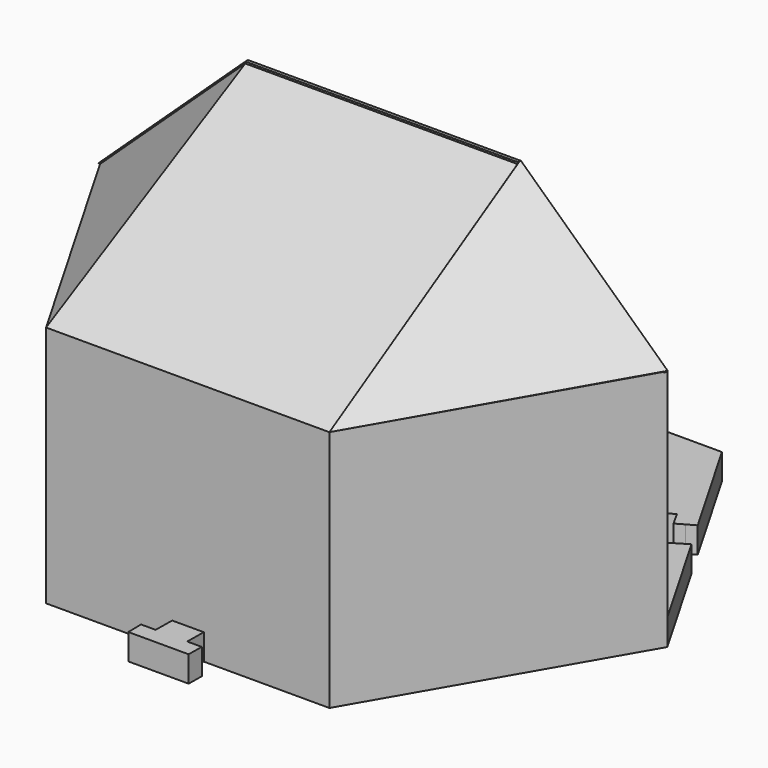
from build123d import *

# Parameters (mm, degrees)
F0_W      = 50
F0_H      = 12.5
F1_DEPTH  = 8
F2_DEPTH  = 75
F4_DEPTH  = 8
F7_DEPTH  = 3
F8_DEPTH  = 1
F11_DEPTH = 3
F14_DEPTH = 3
F15_DEPTH = 8
F16_DEPTH = 25
F17_DEPTH = 8
F18_DEPTH = 8
F19_DEPTH = 8


# Not quite as in the source:
# - a feature names something its author has since deleted; it is built from what else it names


with BuildPart() as f1:
    # F0 (on Top) → F1 (new body)
    with BuildSketch(Plane.XY):
        Polygon((-42.0179491924, 72.7772228311), (-60.5095952989, 40.7487522591), (-57.9695070384, 39.3207329262), (-55.5194165334, 43.6791064608), (-50.2642610162, 40.7248836223), (-52.7144317239, 36.366367418), (-57.615009792, 27.6494680496), (-60.0654171506, 23.2910848888), (-65.3204122546, 26.2455930623), (-62.870004896, 30.6039762231), (-65.5097997054, 32.0881441788), (-84.0358983849, 0), (-42.0179491924, -72.7772228311), (42.0179491924, -72.7772228311), (84.0358983849, 0), (65.5442522784, 32.028470572), (63.0375071287, 30.542699277), (65.5869240764, 26.2416718908), (60.4009142911, 23.1676851313), (60.2621924773, 23.4017175915), (60.0654171506, 23.2910848888), (57.615009792, 27.6494680496), (55.164720758, 32.0079177338), (52.8483970279, 36.1280767392), (52.7526466281, 36.0713280944), (50.2033797707, 40.372634697), (50.3975781651, 40.4877307774), (50.2642610162, 40.7248836223), (55.5194165334, 43.6791064608), (57.9695070384, 39.3207329262), (60.5095952989, 40.7487522591), (42.0179491924, 72.7772228311), align=None)
        with Locations((0, 54.5829171234)):
            Rectangle(F0_W, F0_H, mode=Mode.SUBTRACT)
    extrude(amount=F1_DEPTH)

    # F0 (on Top) → F2 (join)
    with BuildSketch(Plane.XY):
        Polygon((-84.0358983849, 0), (-87.5, 0), (-43.75, -75.7772228311), (-4.799692811, -75.7772228311), (4.9533583678, -75.7772228311), (43.75, -75.7772228311), (87.5, 0), (84.0358983849, 0), (42.0179491924, -72.7772228311), (-42.0179491924, -72.7772228311), align=None)
    extrude(amount=F2_DEPTH)

    # F0 (on Top) → F4 (join)
    with BuildSketch(Plane.XY):
        Polygon((43.75, 75.7772228311), (-43.75, 75.7772228311), (-63.1248363216, 42.2190219338), (-60.5095952989, 40.7487522591), (-42.0179491924, 72.7772228311), (42.0179491924, 72.7772228311), (60.5095952989, 40.7487522591), (63.1248363216, 42.2190219338), align=None)
    extrude(amount=F4_DEPTH)

    # F6 (on face) → F7 (join)
    with BuildSketch(Plane(origin=(0, -50.1312366318, 89.3836679776), x_dir=(1, 0, 0), z_dir=(0, 0.4891706574, -0.872188092))):
        Polygon((43.75, 29.4041920927), (0, 29.4041920927), (-43.75, 29.4041920927), (-42.01795, -57.4775522498), (42.01795, -57.4775522498), align=None)
    extrude(amount=F7_DEPTH)

    # F3 (on Front) → F8 (join)
    with BuildSketch(Plane.XZ):
        Polygon((-42.01795, 114.5), (0, 114.5), (42.01795, 114.5), (84.0359, 75), (87.5, 75), (42.01795, 117.5), (0, 117.5), (-42.01795, 117.5), (-87.5, 75), (-84.0359, 75), align=None)
    extrude(amount=F8_DEPTH)

    # F10 (on face) → F11 (join)
    with BuildSketch(Plane(origin=(-67.6846727043, -39.0777640058, 72.4338274863), x_dir=(0.7723629594, -0.3015876344, 0.5590173143), z_dir=(-0.6351814378, -0.3667221741, 0.6797495039))):
        Polygon((33.2314262259, 55.789645187), (-25.6554603702, 35.6104118215), (30.9888924807, -31.0804218073), align=None)
    extrude(amount=-F11_DEPTH)

    # F13 (on face) → F14 (join)
    with BuildSketch(Plane(origin=(67.6756688636, -39.5950852503, 72.4241918832), x_dir=(0.7733047167, 0.3041472681, -0.556322078), z_dir=(-0.6340345536, 0.3709553614, -0.6785221475))):
        Polygon((-30.939509805, 30.5117392321), (-32.8751652468, -56.3649154418), (25.9400068576, -35.9776056011), align=None)
    extrude(amount=F14_DEPTH)

    # F0 (on Top) → F15 (join)
    with BuildSketch(Plane.XY):
        with Locations((0, 54.5829171234)):
            Rectangle(F0_W, F0_H)
    extrude(amount=F15_DEPTH)

    # F0 (on Top) → F16 (cut)
    with BuildSketch(Plane.XY):
        Polygon((-57.9695070384, 39.3207329262), (-60.5095952989, 40.7487522591), (-65.5097997054, 32.0881441788), (-62.870004896, 30.6039762231), (-57.615009792, 27.6494680496), (-52.7144317239, 36.366367418), align=None)
    extrude(amount=-F16_DEPTH, mode=Mode.SUBTRACT)

    # F0 (on Top) → F17 (join)
    with BuildSketch(Plane.XY):
        Polygon((-65.5097997054, 32.0881441788), (-68.125, 33.5584843966), (-87.5, 0), (-84.0358983849, 0), align=None)
        Polygon((87.5, 0), (68.1251636784, 33.5582008974), (65.5442522784, 32.028470572), (84.0358983849, 0), align=None)
    extrude(amount=F17_DEPTH)

    # F0 (on Top) → F18 (join)
    with BuildSketch(Plane.XY):
        Polygon((4.9533583678, -75.7772228311), (-4.799692811, -75.7772228311), (-4.8760764436, -82.0772228311), (-4.9366983742, -87.0772228311), (-4.8147415831, -87.0772228311), (4.8147415831, -87.0772228311), (4.8760764436, -82.0772228311), align=None)
        Polygon((9.3760764436, -82.0772228311), (4.8760764436, -82.0772228311), (4.8147415831, -87.0772228311), (9.3147415831, -87.0772228311), align=None)
    extrude(amount=F18_DEPTH)

    # F0 (on Top) → F19 (join)
    with BuildSketch(Plane.XY):
        Polygon((-4.9366983742, -87.0772228311), (-4.8760764436, -82.0772228311), (-9.3760764436, -82.0772228311), (-9.3147415831, -87.0772228311), align=None)
    extrude(amount=F19_DEPTH)


solid = f1.part
